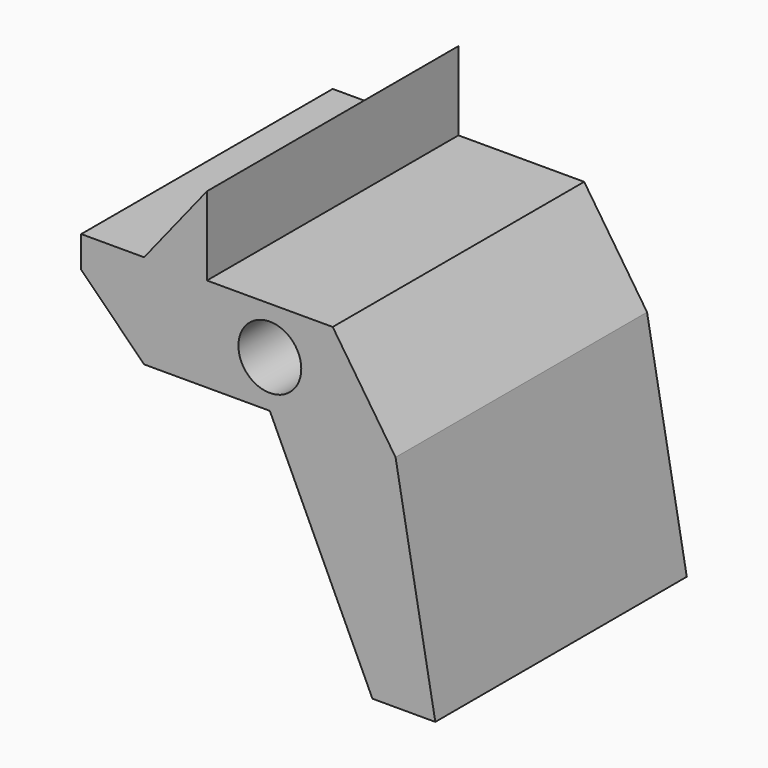
from build123d import *

# Parameters (mm, degrees)
F0_R     = 1.27
F1_DEPTH = 12.7


# Not quite as in the source:
# - a feature names something its author has since deleted; it is built from what else it names


with BuildPart() as f1:
    # F0 (on Front) → F1 (new body)
    with BuildSketch(Plane.XZ):
        Polygon((2.54, -3.81), (0, 0), (-5.08, 0), (-7.62, 0), (-10.16, 0), (-10.16, -1.27), (-7.62, -3.81), (-2.54, -3.81), (1.605475081, -12.7), (4.145475081, -12.7), align=None)
        with Locations((-2.54, -1.905)):
            Circle(F0_R, mode=Mode.SUBTRACT)
        Polygon((-7.62, 0), (-5.08, 0), (-5.08, 3.175), align=None)
    extrude(amount=F1_DEPTH)


solid = f1.part
